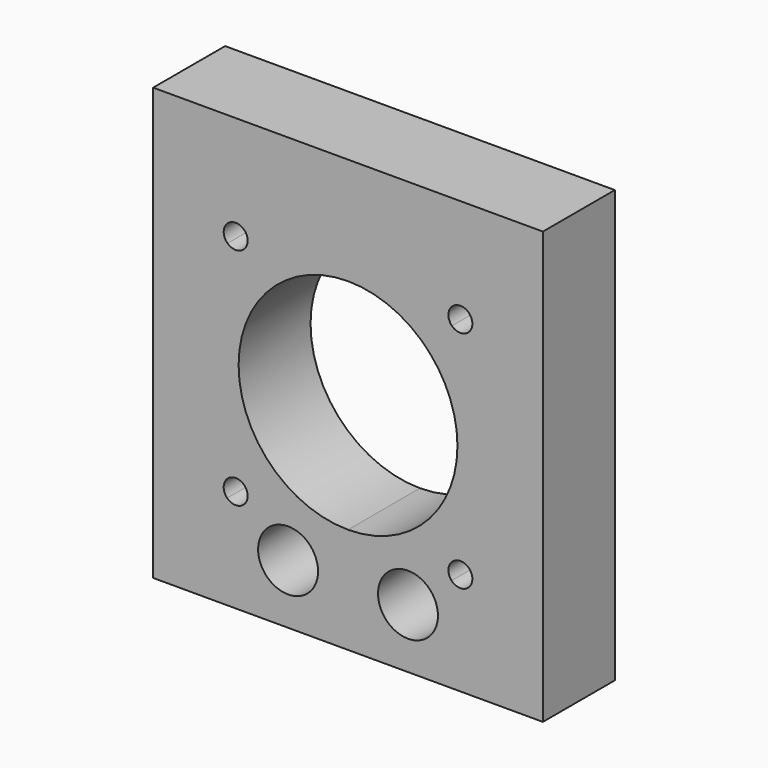
from build123d import *

# Parameters (mm, degrees)
F0_W      = 65
F0_H      = 65
F1_DEPTH  = 15
F3_DEPTH  = 15
F5_DEPTH  = 25
F6_R      = 5
F7_DEPTH  = 11
F8_R      = 2
F9_DEPTH  = 25
F10_R     = 5
F11_DEPTH = 11
F13_DEPTH = 4
F14_R     = 4
F15_DEPTH = 6
F16_DEPTH = 7


# Not quite as in the source:
# - the program builds the solid bodies; features that only make, move or delete a surface that nothing else refers to are left out


with BuildPart() as f1:
    # F0 (on Front) → F1 (new body)
    with BuildSketch(Plane.XZ):
        Rectangle(F0_W, F0_H)
    extrude(amount=F1_DEPTH)

    # F2 (on face) → F3 (cut)
    with BuildSketch(Plane.XZ.offset(15)):
        with BuildLine():
            ThreePointArc((18.25, 3.4), (-12.9046987567, 16.3046987567), (0, -14.85))
            ThreePointArc((0, -14.85), (12.9046987567, -9.5046987567), (18.25, 3.4))
        make_face()
    extrude(amount=-F3_DEPTH, mode=Mode.SUBTRACT)

    # F4 (on face) → F5 (cut)
    with BuildSketch(Plane.XZ.offset(15)):
        with BuildLine():
            ThreePointArc((-20.0981694395, 20.6717568643), (-19.4320900923, 21.4178765299), (-18.7383297014, 22.1383297014))
            Line((-18.7383297014, 22.1383297014), (-20.1525432638, 23.5525432638))
            ThreePointArc((-20.1525432638, 23.5525432638), (-20.7379735443, 22.1005871312), (-20.0981694395, 20.6717568643))
        make_face()
        with BuildLine():
            ThreePointArc((18.7383297014, 22.1383297014), (19.4320900923, 21.4178765299), (20.0981694395, 20.6717568643))
            ThreePointArc((20.0981694395, 20.6717568643), (20.5713162639, 21.338229544), (20.7383297014, 22.1383297014))
            ThreePointArc((20.7383297014, 22.1383297014), (20.5860887665, 22.9036965662), (20.1525432638, 23.5525432638))
            Line((20.1525432638, 23.5525432638), (18.7383297014, 22.1383297014))
        make_face()
        with BuildLine():
            Line((17.3241161391, 20.7241161391), (18.7383297014, 22.1383297014))
            ThreePointArc((18.7383297014, 22.1383297014), (18.0178765299, 22.8320900923), (17.2717568643, 23.4981694395))
            ThreePointArc((17.2717568643, 23.4981694395), (16.7386858586, 22.1005871312), (17.3241161391, 20.7241161391))
        make_face()
        with BuildLine():
            ThreePointArc((17.2717568643, 23.4981694395), (18.0178765299, 22.8320900923), (18.7383297014, 22.1383297014))
            Line((18.7383297014, 22.1383297014), (20.1525432638, 23.5525432638))
            ThreePointArc((20.1525432638, 23.5525432638), (18.7005871312, 24.1379735443), (17.2717568643, 23.4981694395))
        make_face()
        with BuildLine():
            ThreePointArc((17.3241161391, 20.7241161391), (18.7005871312, 20.1386858586), (20.0981694395, 20.6717568643))
            ThreePointArc((20.0981694395, 20.6717568643), (19.4320900923, 21.4178765299), (18.7383297014, 22.1383297014))
            Line((18.7383297014, 22.1383297014), (17.3241161391, 20.7241161391))
        make_face()
        with BuildLine():
            ThreePointArc((20.7383297014, -15.3383297014), (20.5713162639, -14.538229544), (20.0981694395, -13.8717568643))
            ThreePointArc((20.0981694395, -13.8717568643), (19.4320900923, -14.6178765299), (18.7383297014, -15.3383297014))
            Line((18.7383297014, -15.3383297014), (20.1525432638, -16.7525432638))
            ThreePointArc((20.1525432638, -16.7525432638), (20.5860887665, -16.1036965662), (20.7383297014, -15.3383297014))
        make_face()
        with BuildLine():
            ThreePointArc((18.7383297014, -15.3383297014), (19.4320900923, -14.6178765299), (20.0981694395, -13.8717568643))
            ThreePointArc((20.0981694395, -13.8717568643), (18.7005871312, -13.3386858586), (17.3241161391, -13.9241161391))
            Line((17.3241161391, -13.9241161391), (18.7383297014, -15.3383297014))
        make_face()
        with BuildLine():
            Line((20.1525432638, -16.7525432638), (18.7383297014, -15.3383297014))
            ThreePointArc((18.7383297014, -15.3383297014), (18.0178765299, -16.0320900923), (17.2717568643, -16.6981694395))
            ThreePointArc((17.2717568643, -16.6981694395), (18.7005871312, -17.3379735443), (20.1525432638, -16.7525432638))
        make_face()
        with BuildLine():
            ThreePointArc((17.2717568643, -16.6981694395), (18.0178765299, -16.0320900923), (18.7383297014, -15.3383297014))
            Line((18.7383297014, -15.3383297014), (17.3241161391, -13.9241161391))
            ThreePointArc((17.3241161391, -13.9241161391), (16.7386858586, -15.3005871312), (17.2717568643, -16.6981694395))
        make_face()
        with BuildLine():
            ThreePointArc((-18.7383297014, 22.1383297014), (-18.0178765299, 22.8320900923), (-17.2717568643, 23.4981694395))
            ThreePointArc((-17.2717568643, 23.4981694395), (-18.7005871312, 24.1379735443), (-20.1525432638, 23.5525432638))
            Line((-20.1525432638, 23.5525432638), (-18.7383297014, 22.1383297014))
        make_face()
        with BuildLine():
            ThreePointArc((-16.7383297014, 22.1383297014), (-16.8764562264, 22.8686906826), (-17.2717568643, 23.4981694395))
            ThreePointArc((-17.2717568643, 23.4981694395), (-18.0178765299, 22.8320900923), (-18.7383297014, 22.1383297014))
            Line((-18.7383297014, 22.1383297014), (-17.3241161391, 20.7241161391))
            ThreePointArc((-17.3241161391, 20.7241161391), (-16.8905706364, 21.3729628367), (-16.7383297014, 22.1383297014))
        make_face()
        with BuildLine():
            Line((-17.3241161391, 20.7241161391), (-18.7383297014, 22.1383297014))
            ThreePointArc((-18.7383297014, 22.1383297014), (-19.4320900923, 21.4178765299), (-20.0981694395, 20.6717568643))
            ThreePointArc((-20.0981694395, 20.6717568643), (-18.7005871312, 20.1386858586), (-17.3241161391, 20.7241161391))
        make_face()
        with BuildLine():
            ThreePointArc((-18.7383297014, -15.3383297014), (-18.0178765299, -16.0320900923), (-17.2717568643, -16.6981694395))
            ThreePointArc((-17.2717568643, -16.6981694395), (-16.8764562264, -16.0686906826), (-16.7383297014, -15.3383297014))
            ThreePointArc((-16.7383297014, -15.3383297014), (-16.8905706364, -14.5729628367), (-17.3241161391, -13.9241161391))
            Line((-17.3241161391, -13.9241161391), (-18.7383297014, -15.3383297014))
        make_face()
        with BuildLine():
            Line((-20.1525432638, -16.7525432638), (-18.7383297014, -15.3383297014))
            ThreePointArc((-18.7383297014, -15.3383297014), (-19.4320900923, -14.6178765299), (-20.0981694395, -13.8717568643))
            ThreePointArc((-20.0981694395, -13.8717568643), (-20.7379735443, -15.3005871312), (-20.1525432638, -16.7525432638))
        make_face()
        with BuildLine():
            ThreePointArc((-20.1525432638, -16.7525432638), (-18.7005871312, -17.3379735443), (-17.2717568643, -16.6981694395))
            ThreePointArc((-17.2717568643, -16.6981694395), (-18.0178765299, -16.0320900923), (-18.7383297014, -15.3383297014))
            Line((-18.7383297014, -15.3383297014), (-20.1525432638, -16.7525432638))
        make_face()
        with BuildLine():
            ThreePointArc((-20.0981694395, -13.8717568643), (-19.4320900923, -14.6178765299), (-18.7383297014, -15.3383297014))
            Line((-18.7383297014, -15.3383297014), (-17.3241161391, -13.9241161391))
            ThreePointArc((-17.3241161391, -13.9241161391), (-18.7005871312, -13.3386858586), (-20.0981694395, -13.8717568643))
        make_face()
    extrude(amount=-F5_DEPTH, mode=Mode.SUBTRACT)

    # F6 (on face) → F7 (cut)
    with BuildSketch(Plane(origin=(0, 0, 0), x_dir=(-1, 0, 0), z_dir=(0, 1, 0))):
        with Locations((-18.7383297014, 22.1383297014)):
            Circle(F6_R)
        with Locations((18.7383297014, 22.1383297014)):
            Circle(F6_R)
        with Locations((-18.7383297014, -15.3383297014)):
            Circle(F6_R)
        with Locations((18.7383297014, -15.3383297014)):
            Circle(F6_R)
    extrude(amount=-F7_DEPTH, mode=Mode.SUBTRACT)

    # F8 (on face) → F9 (cut)
    with BuildSketch(Plane(origin=(0, 0, 0), x_dir=(-1, 0, 0), z_dir=(0, 1, 0))):
        with BuildLine():
            ThreePointArc((12, -22.6), (10, -20.6), (8, -22.6))
            ThreePointArc((8, -22.6), (10, -24.6), (12, -22.6))
        make_face()
        with Locations((-10, -22.6)):
            Circle(F8_R)
    extrude(amount=-F9_DEPTH, mode=Mode.SUBTRACT)

    # F10 (on face) → F11 (cut)
    with BuildSketch(Plane.XZ.offset(15)):
        with Locations((-10, -22.6)):
            Circle(F10_R)
        with Locations((10, -22.6)):
            Circle(F10_R)
    extrude(amount=-F11_DEPTH, mode=Mode.SUBTRACT)

    # F12 (on face) → F13 (cut)
    with BuildSketch(Plane(origin=(0, 0, -32.5), x_dir=(1, 0, 0), z_dir=(0, 0, -1))):
        with BuildLine():
            ThreePointArc((-8, 2.5), (-11.4142135624, 3.9142135624), (-10, 0.5))
            Line((-10, 0.5), (-10, 2.5))
            Line((-10, 2.5), (-8, 2.5))
        make_face()
        with BuildLine():
            ThreePointArc((12, 2.5), (10, 4.5), (8, 2.5))
            ThreePointArc((8, 2.5), (10, 0.5), (12, 2.5))
        make_face()
        with BuildLine():
            Line((-10, 2.5), (-10, 0.5))
            ThreePointArc((-10, 0.5), (-8.5857864376, 1.0857864376), (-8, 2.5))
            Line((-8, 2.5), (-10, 2.5))
        make_face()
    extrude(amount=-F13_DEPTH, mode=Mode.SUBTRACT)

    # F14 (on face) → F15 (cut)
    with BuildSketch(Plane(origin=(0, 0, 0), x_dir=(-1, 0, 0), z_dir=(0, 1, 0))):
        with Locations((-19, -21.5)):
            Circle(F14_R)
        with BuildLine():
            ThreePointArc((23, -21.5), (19, -17.5), (15, -21.5))
            ThreePointArc((15, -21.5), (19, -25.5), (23, -21.5))
        make_face()
    extrude(amount=-F15_DEPTH, mode=Mode.SUBTRACT)

    # F16 (add): a face of the model
    f16_faces = [f1.faces().sort_by_distance(p)[0] for p in [
        (0, -7.5, 32.5),
    ]]
    extrude(f16_faces, amount=F16_DEPTH)


solid = f1.part
